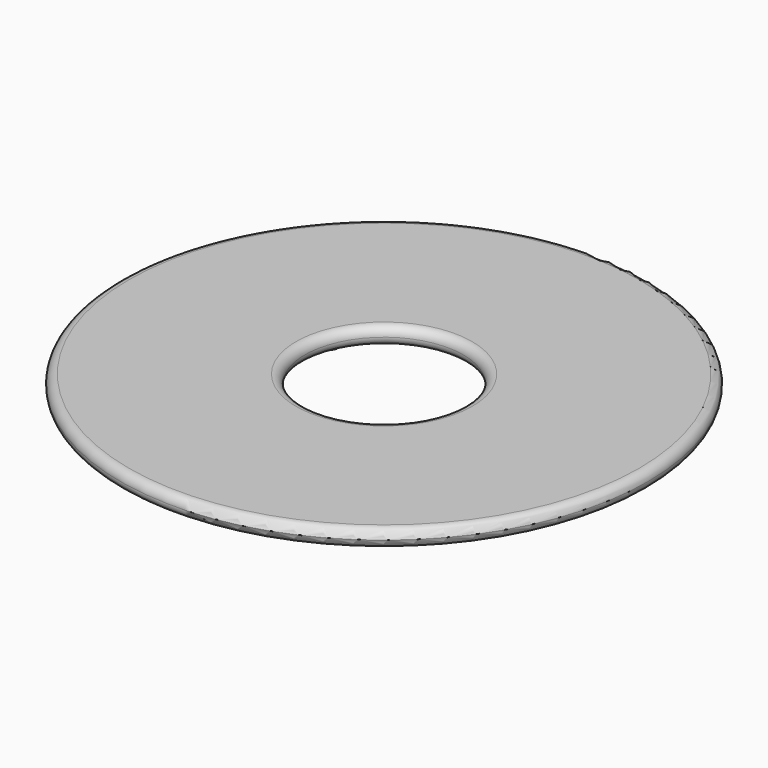
from build123d import *

# Parameters (mm, degrees)
F0_R     = 30
F0_R_2   = 9
F1_DEPTH = 2
F2_R     = 0.99999
F4_DEPTH = 1.5


# Not quite as in the source:
# - a fillet or chamfer is up to 0.001 mm smaller than in the source, because OpenCascade refuses the exact size


with BuildPart() as f1:
    # F0 (on Top) → F1 (new body)
    with BuildSketch(Plane.XY):
        Circle(F0_R)
        Circle(F0_R_2, mode=Mode.SUBTRACT)
    extrude(amount=F1_DEPTH)

    # F2 (radius 1 in the source; OpenCascade refuses exactly that, so slightly less here)
    f2_edges = [f1.edges().sort_by_distance(p)[0] for p in [
        (-9, 0, 2),
        (-9, 0, 0),
        (-30, 0, 0),
        (-30, 0, 2),
    ]]
    fillet(f2_edges, radius=F2_R)


with BuildPart() as f4:
    # F3 (on Top) → F4 (new body)
    with BuildSketch(Plane.XY):
        with BuildLine():
            Line((13.1136951927, 7.9880466137), (13.863694881, 7.9873627843))
            Line((13.863694881, 7.9873627843), (13.4881028232, 7.3381859161))
            ThreePointArc((13.4881028232, 7.3381859161), (14.2383987351, 7.3376728416), (14.613694881, 7.9873627843))
            ThreePointArc((14.613694881, 7.9873627843), (13.8640367957, 8.7373627064), (13.1136951927, 7.9880466137))
        make_face()
        with BuildLine():
            Line((13.4881028232, 7.3381859161), (13.863694881, 7.9873627843))
            Line((13.863694881, 7.9873627843), (13.1136951927, 7.9880466137))
            ThreePointArc((13.1136951927, 7.9880466137), (13.2138341834, 7.6129551538), (13.4881028232, 7.3381859161))
        make_face()
    extrude(amount=-F4_DEPTH)


with BuildPart() as f4b:
    # F3 (on Top) → F4, piece 2 (new body)
    with BuildSketch(Plane.XY):
        with BuildLine():
            Line((10.5142524025, 6.4904160916), (11.2642520908, 6.4897322622))
            Line((11.2642520908, 6.4897322622), (10.888660033, 5.8405553941))
            ThreePointArc((10.888660033, 5.8405553941), (11.638955945, 5.8400423195), (12.0142520908, 6.4897322622))
            ThreePointArc((12.0142520908, 6.4897322622), (11.2645940055, 7.2397321843), (10.5142524025, 6.4904160916))
        make_face()
        with BuildLine():
            Line((10.888660033, 5.8405553941), (11.2642520908, 6.4897322622))
            Line((11.2642520908, 6.4897322622), (10.5142524025, 6.4904160916))
            ThreePointArc((10.5142524025, 6.4904160916), (10.6143913932, 6.1153246317), (10.888660033, 5.8405553941))
        make_face()
    extrude(amount=-F4_DEPTH)


with BuildPart() as f4c:
    # F3 (on Top) → F4, piece 3 (new body)
    with BuildSketch(Plane.XY):
        with BuildLine():
            ThreePointArc((-13.4746988904, 7.3627698675), (-13.1999296527, 7.6370385073), (-13.0991068327, 8.0119467357))
            Line((-13.0991068327, 8.0119467357), (-13.8491065209, 8.0126305651))
            Line((-13.8491065209, 8.0126305651), (-13.4746988904, 7.3627698675))
        make_face()
        with BuildLine():
            Line((-13.8491065209, 8.0126305651), (-13.0991068327, 8.0119467357))
            ThreePointArc((-13.0991068327, 8.0119467357), (-13.0991065989, 8.0122886504), (-13.0991065209, 8.0126305651))
            ThreePointArc((-13.0991065209, 8.0126305651), (-14.4984545489, 8.3879266329), (-13.4746988904, 7.3627698675))
            Line((-13.4746988904, 7.3627698675), (-13.8491065209, 8.0126305651))
        make_face()
    extrude(amount=-F4_DEPTH)


with BuildPart() as f4d:
    # F3 (on Top) → F4, piece 4 (new body)
    with BuildSketch(Plane.XY):
        with BuildLine():
            Line((-11.2523990482, 6.5102623341), (-10.50239936, 6.5095785047))
            ThreePointArc((-10.50239936, 6.5095785047), (-10.5023991262, 6.5099204194), (-10.5023990482, 6.5102623341))
            ThreePointArc((-10.5023990482, 6.5102623341), (-11.9017470762, 6.885558402), (-10.8779914177, 5.8604016366))
            Line((-10.8779914177, 5.8604016366), (-11.2523990482, 6.5102623341))
        make_face()
        with BuildLine():
            ThreePointArc((-10.8779914177, 5.8604016366), (-10.6032221801, 6.1346702764), (-10.50239936, 6.5095785047))
            Line((-10.50239936, 6.5095785047), (-11.2523990482, 6.5102623341))
            Line((-11.2523990482, 6.5102623341), (-10.8779914177, 5.8604016366))
        make_face()
    extrude(amount=-F4_DEPTH)


with BuildPart() as f4e:
    # F3 (on Top) → F4, piece 5 (new body)
    with BuildSketch(Plane.XY):
        with BuildLine():
            ThreePointArc((0.7381469575, -12.9999945964), (0.6378369002, -12.6252907422), (0.3637390152, -12.3508177282))
            Line((0.3637390152, -12.3508177282), (-0.0118530425, -12.9999945964))
            Line((-0.0118530425, -12.9999945964), (-0.386260673, -12.3501338988))
            ThreePointArc((-0.386260673, -12.3501338988), (-0.3871491104, -13.6493426243), (0.7381469575, -12.9999945964))
        make_face()
        with BuildLine():
            Line((-0.0118530425, -12.9999945964), (0.3637390152, -12.3508177282))
            ThreePointArc((0.3637390152, -12.3508177282), (-0.0111692132, -12.2499949081), (-0.386260673, -12.3501338988))
            Line((-0.386260673, -12.3501338988), (-0.0118530425, -12.9999945964))
        make_face()
    extrude(amount=-F4_DEPTH)


with BuildPart() as f4f:
    # F3 (on Top) → F4, piece 6 (new body)
    with BuildSketch(Plane.XY):
        with BuildLine():
            Line((-0.01458836, -15.9999933494), (0.3610036977, -15.3508164812))
            ThreePointArc((0.3610036977, -15.3508164812), (-0.0139045307, -15.2499936611), (-0.3889959906, -15.3501326518))
            Line((-0.3889959906, -15.3501326518), (-0.01458836, -15.9999933494))
        make_face()
        with BuildLine():
            ThreePointArc((0.73541164, -15.9999933494), (0.6351015827, -15.6252894952), (0.3610036977, -15.3508164812))
            Line((0.3610036977, -15.3508164812), (-0.01458836, -15.9999933494))
            Line((-0.01458836, -15.9999933494), (-0.3889959906, -15.3501326518))
            ThreePointArc((-0.3889959906, -15.3501326518), (-0.3898844279, -16.6493413773), (0.73541164, -15.9999933494))
        make_face()
    extrude(amount=-F4_DEPTH)


solid = Compound([f1.part, f4.part, f4b.part, f4c.part, f4d.part, f4e.part, f4f.part])
